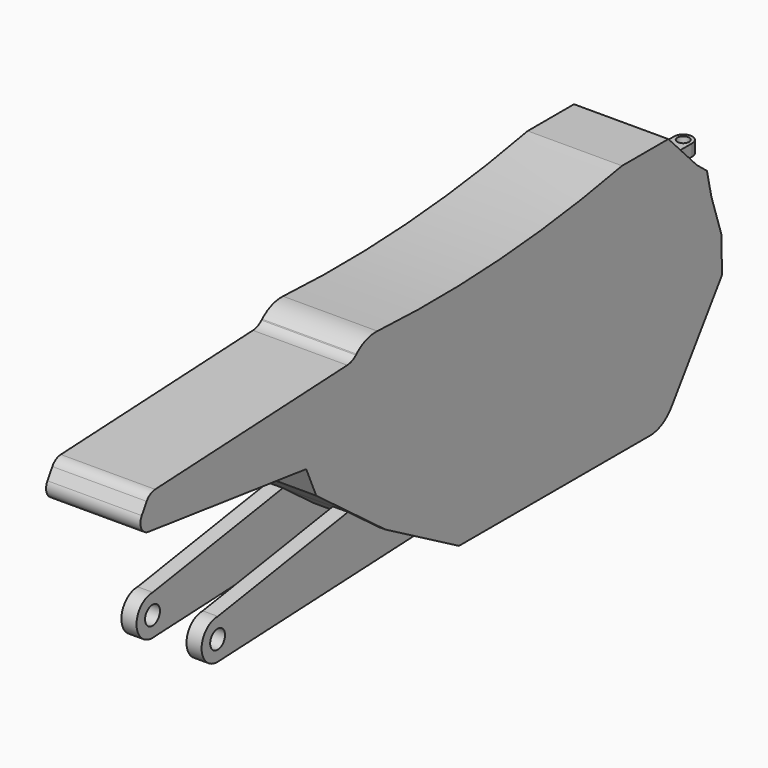
from build123d import *

# Parameters (mm, degrees)
F1_DEPTH      = 5.08
F1_DEPTH_BACK = 5.08
F2_START      = 2.6924
F0_R          = 1.0003723125
F2_DEPTH      = 1.6256
F5_START      = 9.652
F4_R          = 0.635
F5_DEPTH      = 1.27
F6_START      = 6.35
F6_DEPTH      = 1.27


with BuildPart() as f1:
    # F0 (on Right) → F1 (new body, two sides)
    with BuildSketch(Plane.YZ) as f1_sk:
        with BuildLine():
            Line((0.0852813464, 0.1919296192), (0.0287976927, 4.0513155982))
            Line((0.0287976927, 4.0513155982), (-1.336822079, 8.2203539118))
            Line((-1.336822079, 8.2203539118), (-1.9315851387, 10.914305225))
            Line((-1.9315851387, 10.914305225), (-3.2904522843, 12.013522602))
            Line((-3.2904522843, 12.013522602), (-7.1285278888, 16.0394304962))
            Line((-7.1285278888, 16.0394304962), (-13.3653870204, 16.0394304962))
            ThreePointArc((-13.3653870204, 16.0394304962), (-29.7626529342, 13.8664815487), (-46.3029045757, 13.7564260577))
            ThreePointArc((-46.3029045757, 13.7564260577), (-47.8190863835, 13.5325193665), (-49.1243677886, 12.7292871869))
            Line((-49.1243677886, 12.7292871869), (-49.1957577746, 12.6622238566))
            ThreePointArc((-49.1957577746, 12.6622238566), (-49.7319383294, 12.3126553679), (-50.3558819852, 12.1698897204))
            Line((-50.3558819852, 12.1698897204), (-76.2232715204, 10.9134739549))
            ThreePointArc((-76.2232715204, 10.9134739549), (-76.8763540697, 10.7170137111), (-77.3614025915, 10.237595965))
            Line((-77.3614025915, 10.237595965), (-78.0212117411, 9.1555053464))
            ThreePointArc((-78.0212117411, 9.1555053464), (-78.1109393732, 8.0141207108), (-77.2434551545, 7.2669386283))
            Line((-77.2434551545, 7.2669386283), (-55.8863058686, 4.5678056777))
            Line((-55.8863058686, 4.5678056777), (-54.5319553308, 1.4966176624))
            Line((-54.5319553308, 1.4966176624), (-49.3058934109, -2.4282623857))
            Line((-49.3058934109, -2.4282623857), (-45.1969819986, -5.514139413))
            Line((-45.1969819986, -5.514139413), (-40.2585836646, -8.2946047065))
            Line((-40.2585836646, -8.2946047065), (-35.3201853305, -11.07507))
            Line((-35.3201853305, -11.07507), (-9.6430980807, -11.07507))
            ThreePointArc((-9.6430980807, -11.07507), (-7.9967951351, -10.6717705814), (-6.7233083962, -9.5532021501))
            Line((-6.7233083962, -9.5532021501), (0.0852813464, 0.1919296192))
        make_face()
    extrude(amount=F1_DEPTH)
    extrude(f1_sk.sketch, amount=-F1_DEPTH_BACK)

    # F4 (on Top) → F5 (join)
    with BuildSketch(Plane.XY.offset(F5_START)):
        with BuildLine():
            Line((-0.9820741736, 1.1704666201), (-0.9820741736, -1.900618134))
            Line((-0.9820741736, -1.900618134), (0.9820741736, -1.900618134))
            Line((0.9820741736, -1.900618134), (0.9820741736, 1.1704666201))
            Line((0.9820741736, 1.1704666201), (0.9800161632, 1.1704666201))
            ThreePointArc((0.9800161632, 1.1704666201), (0, 2.2146743084), (-0.9800161632, 1.1704666201))
            Line((-0.9800161632, 1.1704666201), (-0.9820741736, 1.1704666201))
        make_face()
        with Locations((0, 1.2326850933)):
            Circle(F4_R, mode=Mode.SUBTRACT)
    extrude(amount=F5_DEPTH)

    # F4 (on Top) → F6 (join)
    with BuildSketch(Plane.XY.offset(F6_START)):
        with BuildLine():
            Line((-0.9820741736, 1.1704666201), (-0.9820741736, -1.900618134))
            Line((-0.9820741736, -1.900618134), (0.9820741736, -1.900618134))
            Line((0.9820741736, -1.900618134), (0.9820741736, 1.1704666201))
            Line((0.9820741736, 1.1704666201), (0.9800161632, 1.1704666201))
            ThreePointArc((0.9800161632, 1.1704666201), (0, 2.2146743084), (-0.9800161632, 1.1704666201))
            Line((-0.9800161632, 1.1704666201), (-0.9820741736, 1.1704666201))
        make_face()
        with Locations((0, 1.2326850933)):
            Circle(F4_R, mode=Mode.SUBTRACT)
    extrude(amount=F6_DEPTH)


with BuildPart() as f2:
    # F0 (on Right) → F2 (new body)
    with BuildSketch(Plane.YZ.offset(F2_START)):
        with BuildLine():
            Line((-66.5820820244, -9.489505192), (-40.2585836646, -8.2946047065))
            Line((-40.2585836646, -8.2946047065), (-45.1969819986, -5.514139413))
            Line((-45.1969819986, -5.514139413), (-49.3058934109, -2.4282623857))
            Line((-49.3058934109, -2.4282623857), (-66.8277770233, -5.1970989376))
            ThreePointArc((-66.8277770233, -5.1970989376), (-69.0123388798, -7.4753769211), (-66.5820820244, -9.489505192))
        make_face()
        with Locations((-66.8605044484, -7.3522070888)):
            Circle(F0_R, mode=Mode.SUBTRACT)
    extrude(amount=F2_DEPTH)


with BuildPart() as f3_1:
    # F3: instance of F2
    add(f2.part.mirror(Plane.YZ))


solid = Compound([f1.part, f2.part, f3_1.part])
